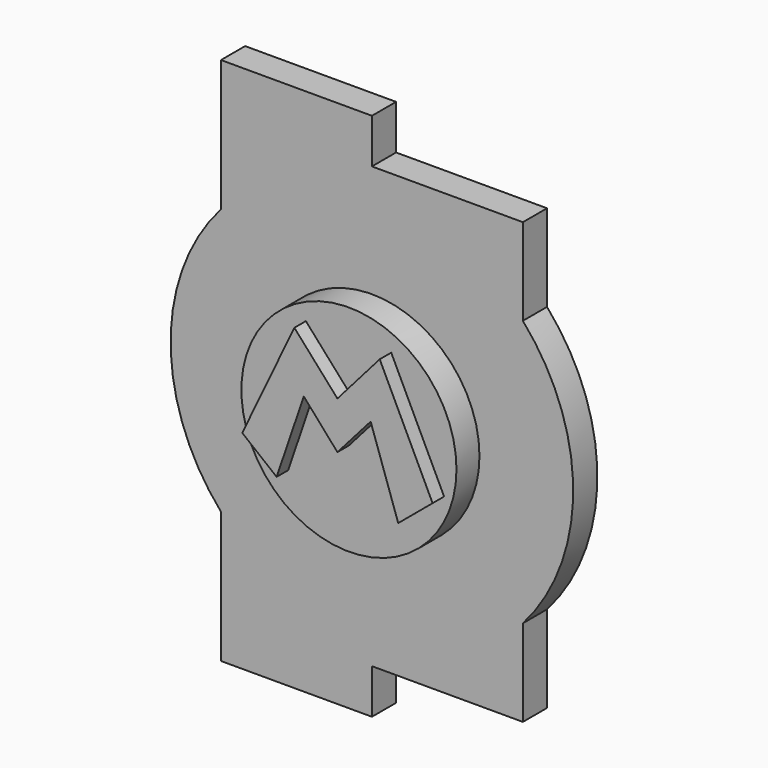
from build123d import *

# Parameters (mm, degrees)
F1_DEPTH = 2.1
F3_DEPTH = 3
F2_R     = 7.4807460639
F4_DEPTH = 2


# Not quite as in the source:
# - a feature names something its author has since deleted; it is built from what else it names


with BuildPart() as f1:
    # F0 (on Front) → F1 (new body)
    with BuildSketch(Plane.XZ):
        with BuildLine():
            Line((0, 15.3), (0, 18.4))
            Line((0, 18.4), (-10.5, 18.4))
            Line((-10.5, 18.4), (-10.5, 9.2601295887))
            ThreePointArc((-10.5, 9.2601295887), (-14, 0), (-10.5, -9.2601295887))
            Line((-10.5, -9.2601295887), (-10.5, -18.4))
            Line((-10.5, -18.4), (0, -18.4))
            Line((0, -18.4), (0, -15.3))
            Line((0, -15.3), (10.5, -15.3))
            Line((10.5, -15.3), (10.5, -9.2601295887))
            ThreePointArc((10.5, -9.2601295887), (14, 0), (10.5, 9.2601295887))
            Line((10.5, 9.2601295887), (10.5, 15.3))
            Line((10.5, 15.3), (0, 15.3))
        make_face()
    extrude(amount=F1_DEPTH)

    # F2 (on face) → F3 (join)
    with BuildSketch(Plane.XZ.offset(2.1)):
        Polygon((-2.9942439869, 5.6681009009), (-6.6190003417, -1.9491401035), (-4.228762351, -3.8665838074), (-2.3375852033, 1.6756160185), (0, -0.9772852063), (2.3115586955, 1.6493498115), (4.2290021665, -3.9453827776), (6.6192396916, -1.9491401035), (2.9419509228, 5.6681009009), (0, 2.3060084786), align=None)
    extrude(amount=F3_DEPTH)

    # F2 (on face) → F4 (join)
    with BuildSketch(Plane.XZ.offset(2.1)):
        Circle(F2_R)
        Polygon((-4.228762351, -3.8665838074), (-6.6190003417, -1.9491401035), (-2.9942439869, 5.6681009009), (0, 2.3060084786), (2.9419509228, 5.6681009009), (6.6192396916, -1.9491401035), (4.2290021665, -3.9453827776), (2.3115586955, 1.6493498115), (0, -0.9772852063), (-2.3375852033, 1.6756160185), align=None, mode=Mode.SUBTRACT)
    extrude(amount=F4_DEPTH)


solid = f1.part
